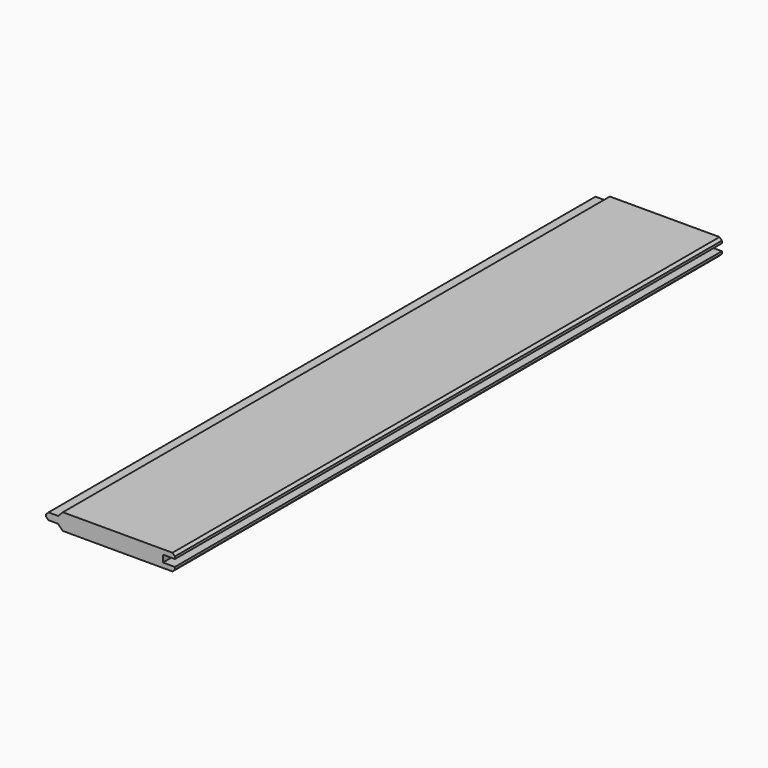
from build123d import *

# Parameters (mm, degrees)
F1_DEPTH = 723.9
F2_SIZE  = 2.54
F3_SIZE  = 5.07999


# Not quite as in the source:
# - a fillet or chamfer is up to 0.001 mm smaller than in the source, because OpenCascade refuses the exact size


with BuildPart() as f1:
    # F0 (on Front) → F1 (new body)
    with BuildSketch(Plane.XZ):
        Polygon((68.199, 3.6576), (68.199, 8.7376), (-55.499, 8.7376), (-55.499, 3.6576), (-68.199, 3.6576), (-68.199, -3.6576), (-55.499, -3.6576), (-55.499, -8.7376), (68.199, -8.7376), (68.199, -3.6576), (55.499, -3.6576), (55.499, 3.6576), align=None)
    extrude(amount=F1_DEPTH)

    # F2
    f2_edges = [f1.edges().sort_by_distance(p)[0] for p in [
        (68.199, -361.95, 8.7376),
        (68.199, -361.95, -8.7376),
        (-68.199, -361.95, 3.6576),
        (-68.199, -361.95, -3.6576),
    ]]
    chamfer(f2_edges, length=F2_SIZE)

    # F3 (size 5.08 in the source; OpenCascade refuses exactly that, so slightly less here)
    f3_edges = [f1.edges().sort_by_distance(p)[0] for p in [
        (-55.499, -361.95, 8.7376),
        (-55.499, -361.95, -8.7376),
    ]]
    chamfer(f3_edges, length=F3_SIZE)


solid = f1.part
